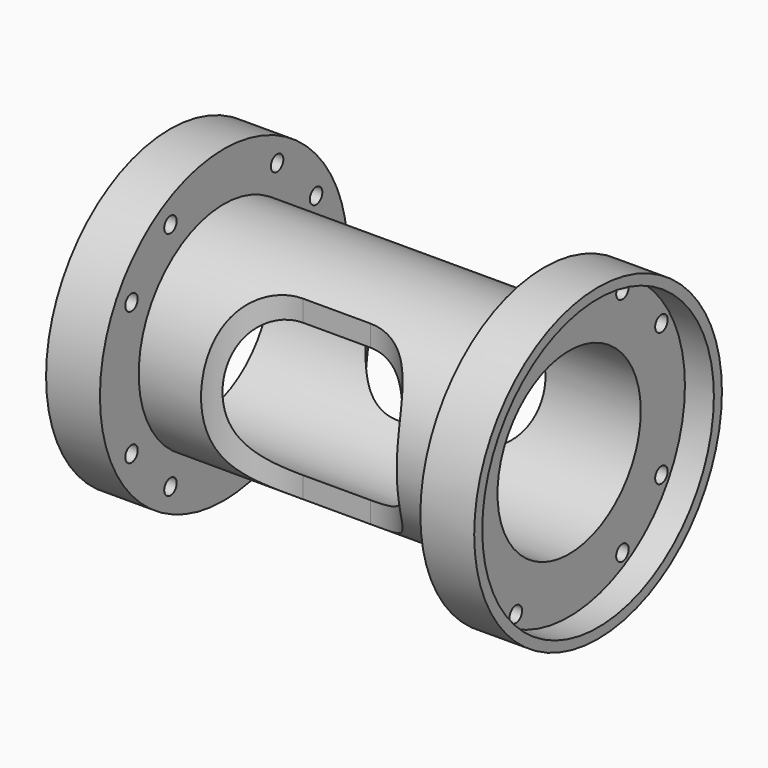
from build123d import *

# Parameters (mm, degrees)
F0_R          = 20.066
F1_DEPTH      = 30.226
F1_DEPTH_BACK = 30.226
F2_R          = 29.21
F2_R_2        = 20.066
F3_DEPTH      = 10.16
F4_R          = 29.21
F4_R_2        = 20.066
F5_DEPTH      = 10.16
F6_R          = 27.31135
F7_DEPTH      = 5.461
F8_R          = 27.31135
F9_DEPTH      = 5.461
F10_R         = 16.891
F11_DEPTH     = 75.312
F12_R         = 1.4732
F13_DEPTH     = 75.312
F16_DEPTH     = 49.277


with BuildPart() as f1:
    # F0 (on Right) → F1 (new body, two sides)
    with BuildSketch(Plane.YZ) as f1_sk:
        Circle(F0_R)
    extrude(amount=F1_DEPTH)
    extrude(f1_sk.sketch, amount=-F1_DEPTH_BACK)

    # F2 (on face) → F3 (join)
    with BuildSketch(Plane.YZ.offset(30.226)):
        Circle(F2_R)
        Circle(F2_R_2, mode=Mode.SUBTRACT)
        Circle(F2_R_2)
    extrude(amount=F3_DEPTH)

    # F4 (on face) → F5 (join)
    with BuildSketch(Plane(origin=(-30.226, 0, 0), x_dir=(0, -1, 0), z_dir=(-1, 0, 0))):
        Circle(F4_R)
        Circle(F4_R_2, mode=Mode.SUBTRACT)
        Circle(F4_R_2)
    extrude(amount=F5_DEPTH)

    # F6 (on face) → F7 (cut)
    with BuildSketch(Plane(origin=(-40.386, 0, 0), x_dir=(0, -1, 0), z_dir=(-1, 0, 0))):
        Circle(F6_R)
    extrude(amount=-F7_DEPTH, mode=Mode.SUBTRACT)

    # F8 (on face) → F9 (cut)
    with BuildSketch(Plane.YZ.offset(40.386)):
        Circle(F8_R)
    extrude(amount=-F9_DEPTH, mode=Mode.SUBTRACT)

    # F10 (on face) → F11 (cut, through all)
    with BuildSketch(Plane.YZ.offset(34.925)):
        Circle(F10_R)
    extrude(amount=-F11_DEPTH, mode=Mode.SUBTRACT)

    # F12 (on face) → F13 (cut, through all)
    with BuildSketch(Plane.YZ.offset(34.925)):
        with Locations((-21.7678, 12.573)):
            Circle(F12_R)
        with Locations((-12.573, 21.7678)):
            Circle(F12_R)
        with Locations((12.573, 21.7678)):
            Circle(F12_R)
        with Locations((21.7678, 12.573)):
            Circle(F12_R)
        with Locations((21.7678, -12.573)):
            Circle(F12_R)
        with Locations((12.573, -21.7678)):
            Circle(F12_R)
        with Locations((-12.573, -21.7678)):
            Circle(F12_R)
        with Locations((-21.7678, -12.573)):
            Circle(F12_R)
    extrude(amount=-F13_DEPTH, mode=Mode.SUBTRACT)

    # F15 (on offset) → F16 (cut, through all)
    with BuildSketch(Plane.XY.offset(20.066)):
        with BuildLine():
            Line((19.05, 30.226), (-19.05, 30.226))
            Line((-19.05, 30.226), (-19.05, 23.876))
            ThreePointArc((-19.05, 23.876), (-15.3302561211, 14.8957438789), (-6.35, 11.176))
            Line((-6.35, 11.176), (6.35, 11.176))
            ThreePointArc((6.35, 11.176), (15.3302561211, 14.8957438789), (19.05, 23.876))
            Line((19.05, 23.876), (19.05, 30.226))
        make_face()
        with BuildLine():
            Line((6.35, -11.176), (-6.35, -11.176))
            ThreePointArc((-6.35, -11.176), (-15.3302561211, -14.8957438789), (-19.05, -23.876))
            Line((-19.05, -23.876), (-19.05, -30.226))
            Line((-19.05, -30.226), (19.05, -30.226))
            Line((19.05, -30.226), (19.05, -23.876))
            ThreePointArc((19.05, -23.876), (15.3302561211, -14.8957438789), (6.35, -11.176))
        make_face()
    extrude(amount=-F16_DEPTH, mode=Mode.SUBTRACT)


solid = f1.part
